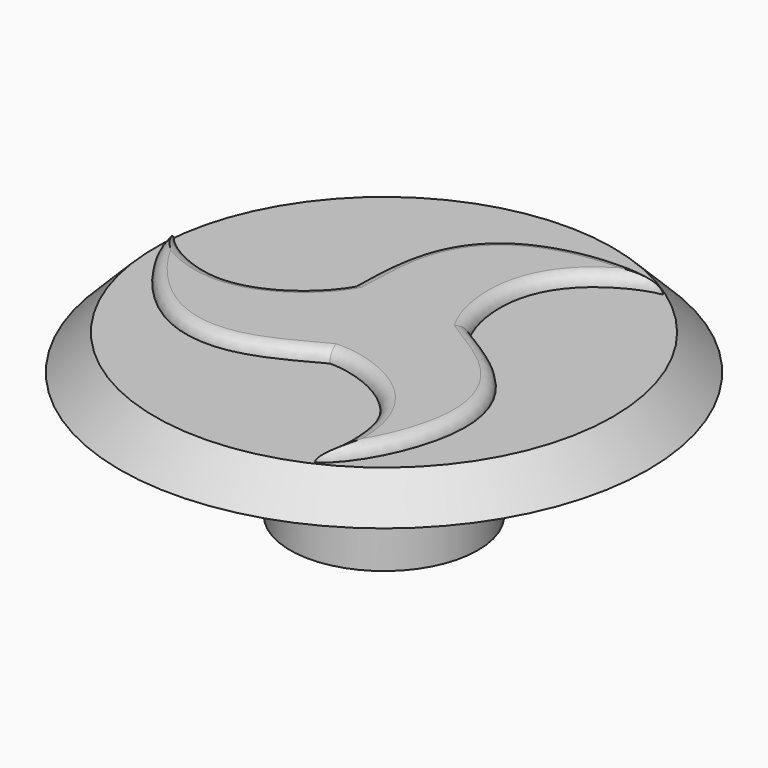
from build123d import *

# Parameters (mm, degrees)
F0_R          = 4.064
F1_DEPTH      = 4.318
F1_DEPTH_BACK = 1.905
F3_START      = 3.556
F2_R          = 11.43
F3_DEPTH      = 1.524
F5_DEPTH      = 0.508
F6_R          = 0.507
F7_SIZE       = 1.52399
F8_R          = 5.334
F8_R_2        = 4.064
F9_DEPTH      = 1.905


# Not quite as in the source:
# - a fillet or chamfer is up to 0.001 mm smaller than in the source, because OpenCascade refuses the exact size


with BuildPart() as f1:
    # F0 (on Top) → F1 (new body, two sides)
    with BuildSketch(Plane.XY) as f1_sk:
        Circle(F0_R)
    extrude(amount=F1_DEPTH)
    extrude(f1_sk.sketch, amount=-F1_DEPTH_BACK)

    # F2 (on Top) → F3 (join)
    with BuildSketch(Plane.XY.offset(F3_START)):
        Circle(F2_R)
    extrude(amount=F3_DEPTH)

    # F4 (on face) → F5 (join)
    with BuildSketch(Plane.XY.offset(5.08)):
        with BuildLine():
            add(Edge.make_bspline(
                [(-2.5404405743, 1.4668987172), (-2.4996633197, 2.1202865286), (-2.6010915613, 5.0110732091), (-0.0142646968, 8.3122067633), (4.3918330124, 8.626762345), (5.6437043386, 8.0404432379)],
                knots=[0, 0, 0, 0, 0.2942307022, 0.6248481818, 1, 1, 1, 1], degree=3))
            add(Edge.make_bspline(
                [(-9.7853695785, 0.8683948085), (-9.2871136075, 0.2474960336), (-7.3361518329, -0.9967433296), (-4.56310729, -0.7262956729), (-2.9385722458, 0.7534186289), (-2.5404405743, 1.4668987172)],
                knots=[0, 0, 0, 0, 0.3382046926, 0.6662572773, 1, 1, 1, 1], degree=3))
            add(Edge.make_bspline(
                [(-0.0004405743, -2.932510334), (-0.5866796448, -3.2238901013), (-3.0394602262, -4.7571228754), (-7.1917391777, -4.1674318727), (-9.6672011569, -0.5089171158), (-9.7853695785, 0.8683948085)],
                knots=[0, 0, 0, 0, 0.2942307022, 0.6248481818, 1, 1, 1, 1], degree=3))
            add(Edge.make_bspline(
                [(4.1403435171, -8.9075509459), (4.4289296438, -8.1655992299), (4.5309916534, -5.8538970897), (2.9102548408, -3.5875938981), (0.8165171431, -2.9205624314), (-0.0004405743, -2.932510334)],
                knots=[0, 0, 0, 0, 0.3382046926, 0.6662572773, 1, 1, 1, 1], degree=3))
            add(Edge.make_bspline(
                [(2.5395594257, 1.4668987172), (3.0850212416, 1.1048906732), (5.6392300646, -0.2526632332), (7.2046821516, -4.1434877901), (5.2740464217, -8.1165581287), (4.1403435171, -8.9075509459)],
                knots=[0, 0, 0, 0, 0.2942307022, 0.6248481818, 1, 1, 1, 1], degree=3))
            add(Edge.make_bspline(
                [(5.6437043386, 8.0404432379), (4.8568622408, 7.9193902968), (2.8038384566, 6.8519275198), (1.6515307263, 4.3151766715), (2.1207333798, 2.168430903), (2.5395594257, 1.4668987172)],
                knots=[0, 0, 0, 0, 0.3382046926, 0.6662572773, 1, 1, 1, 1], degree=3))
        make_face()
    extrude(amount=F5_DEPTH)

    # F6 (radius 0.508 in the source; OpenCascade refuses exactly that, so slightly less here)
    f6_edges = [f1.edges().sort_by_distance(p)[0] for p in [
        (-0.45383, 7.208405, 5.588),
        (2.320924, 5.585189, 5.588),
        (6.468544, -3.210912, 5.588),
        (3.675421, -4.802312, 5.588),
        (-6.016036, -3.996206, 5.588),
        (-5.997667, -0.78159, 5.588),
    ]]
    fillet(f6_edges, radius=F6_R)

    # F7 (size 1.524 in the source; OpenCascade refuses exactly that, so slightly less here)
    f7_edges = [f1.edges().sort_by_distance(p)[0] for p in [
        (-11.43, 0, 5.08),
    ]]
    chamfer(f7_edges, length=F7_SIZE)

    # F8 (on face) → F9 (join)
    with BuildSketch(Plane(origin=(0, 0, 3.556), x_dir=(1, 0, 0), z_dir=(0, 0, -1))):
        Circle(F8_R)
        Circle(F8_R_2, mode=Mode.SUBTRACT)
    extrude(amount=F9_DEPTH)


solid = f1.part
